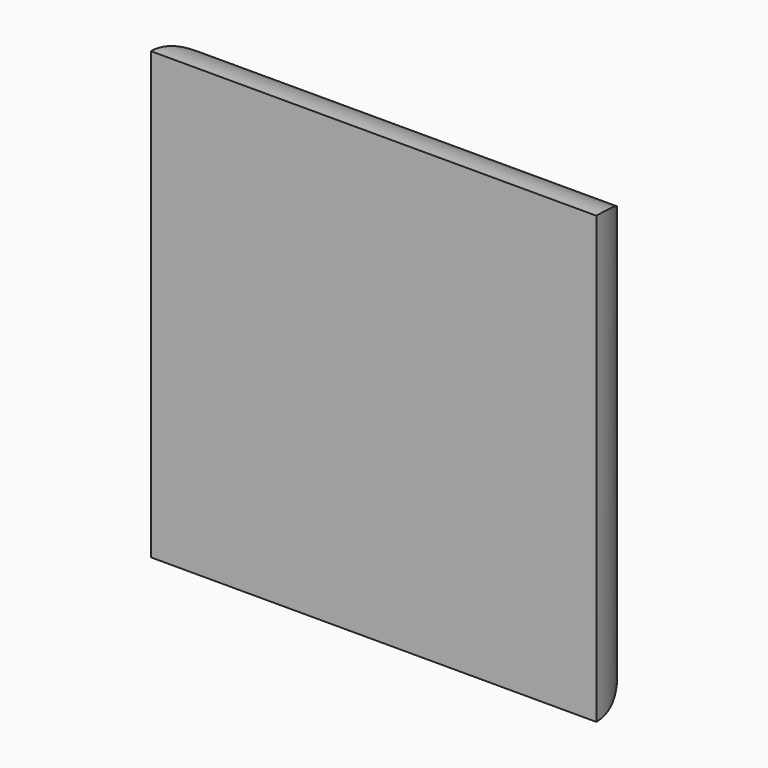
from build123d import *

# Parameters (mm, degrees)
F0_W     = 152.4
F0_H     = 152.4
F1_DEPTH = 25.4
F2_R     = 25.39999


# Not quite as in the source:
# - a fillet or chamfer is up to 0.001 mm smaller than in the source, because OpenCascade refuses the exact size


with BuildPart() as f1:
    # F0 (on Front) → F1 (new body)
    with BuildSketch(Plane.XZ):
        with Locations((-3.7889622442, 0)):
            Rectangle(F0_W, F0_H)
    extrude(amount=F1_DEPTH)

    # F2 (radius 25.4 in the source; OpenCascade refuses exactly that, so slightly less here)
    f2_edges = [f1.edges().sort_by_distance(p)[0] for p in [
        (72.411038, 0, 0),
        (-3.788962, 0, 76.2),
        (-79.988962, 0, 0),
        (-3.788962, 0, -76.2),
    ]]
    fillet(f2_edges, radius=F2_R)


solid = f1.part
